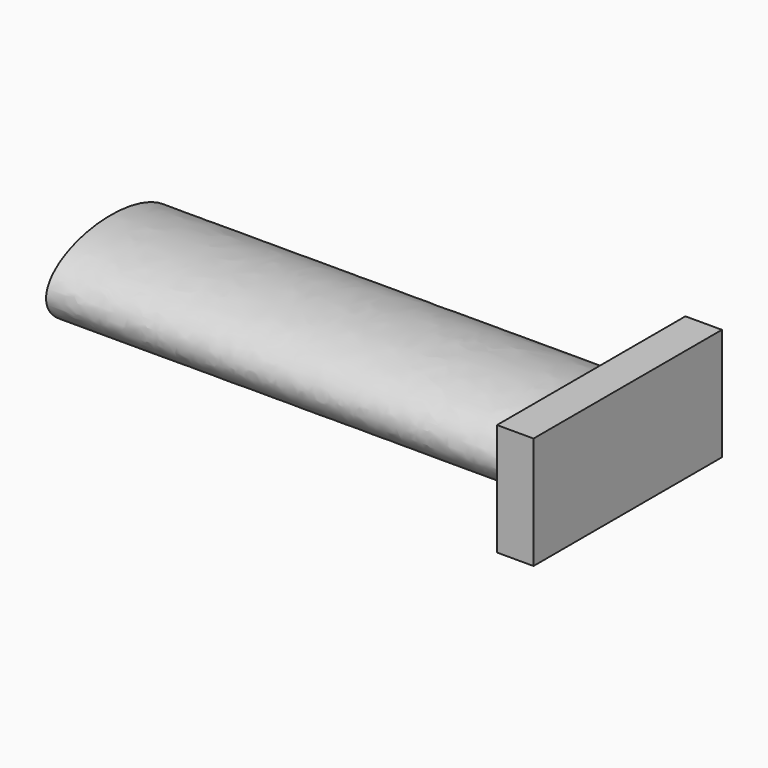
from build123d import *

# Parameters (mm, degrees)
F1_W     = 62.230002135
F1_H     = 29.6578705311
F2_DEPTH = 9.652
F0_W     = 62.230002135
F0_H     = 29.6578705311
F4_DEPTH = 127


# Not quite as in the source:
# - the program builds the solid bodies; features that only make, move or delete a surface that nothing else refers to are left out


with BuildPart() as f2:
    # F1 (on face) → F2 (new body)
    with BuildSketch(Plane.YZ):
        with Locations((0, -58.8321909308)):
            Rectangle(F1_W, F1_H)
    extrude(amount=F2_DEPTH)


with BuildPart() as f2b:
    # F0 (on Right) → F2, piece 2 (new body)
    with BuildSketch(Plane.YZ):
        with Locations((0, -58.8321909308)):
            Rectangle(F0_W, F0_H)
    extrude(amount=F2_DEPTH)


with BuildPart() as f4:
    # F3 (on face) → F4 (new body)
    with BuildSketch(Plane(origin=(0, 0, 0), x_dir=(0, -1, 0), z_dir=(-1, 0, 0))):
        with BuildLine():
            add(Edge.make_bspline(
                [(-21.3132053614, -59.8365403712), (-21.3132053614, -78.3932916774), (10.6566026807, -69.1149160243), (42.6264107227, -59.8365403712), (10.6566026807, -50.558164718), (-21.3132053614, -41.2797890649), (-21.3132053614, -59.8365403712)],
                knots=[0, 0, 0, 2.0943951024, 2.0943951024, 4.1887902048, 4.1887902048, 6.2831853072, 6.2831853072, 6.2831853072], degree=2, weights=[1, 0.5, 1, 0.5, 1, 0.5, 1]))
        make_face()
    extrude(amount=F4_DEPTH)


solid = Compound([f2.part, f2b.part, f4.part])
